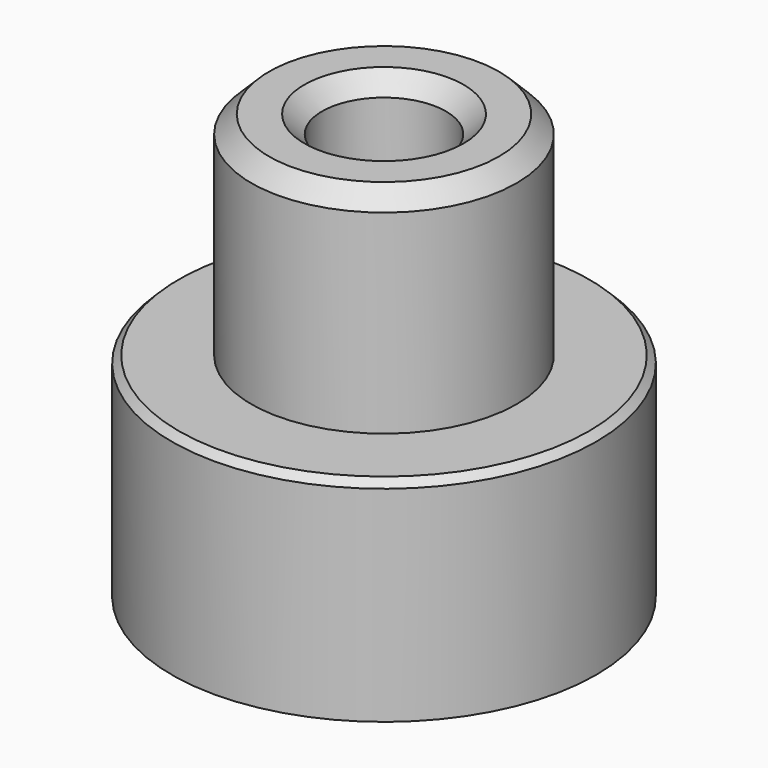
from build123d import *

# Parameters (mm, degrees)
F0_R        = 3.75
F0_R_2      = 1.75
F0_R_3      = 0.9
F1_DEPTH    = 6
F0_R_4      = 6
F1_FACE_R   = 3.75
F1_FACE_R_2 = 0.9
F2_DEPTH    = 6
F3_START    = 8
F3_DEPTH    = 6
F4_SIZE     = 0.5
F5_SIZE     = 0.2
F6_SIZE     = 0.5


with BuildPart() as f1:
    # F0 (on Top) → F1 (new body)
    with BuildSketch(Plane.XY):
        Circle(F0_R)
        Circle(F0_R_2, mode=Mode.SUBTRACT)
        Circle(F0_R_2)
        Circle(F0_R_3, mode=Mode.SUBTRACT)
    extrude(amount=F1_DEPTH)

    # F0 (on Top) + F1_face (on face) → F2 (join)
    with BuildSketch(Plane.XY):
        Circle(F0_R_4)
        Circle(F0_R, mode=Mode.SUBTRACT)
    with BuildSketch(Plane.XY.offset(6)):
        Circle(F1_FACE_R)
        Circle(F1_FACE_R_2, mode=Mode.SUBTRACT)
    extrude(amount=F2_DEPTH)

    # F0 (on Top) → F3 (cut)
    with BuildSketch(Plane.XY.offset(F3_START)):
        Circle(F0_R_2)
        Circle(F0_R_3, mode=Mode.SUBTRACT)
    extrude(amount=F3_DEPTH, mode=Mode.SUBTRACT)

    # F4
    f4_edges = [f1.edges().sort_by_distance(p)[0] for p in [
        (-0.9, 0, 0),
    ]]
    chamfer(f4_edges, length=F4_SIZE)

    # F5
    f5_edges = [f1.edges().sort_by_distance(p)[0] for p in [
        (-6, 0, 6),
    ]]
    chamfer(f5_edges, length=F5_SIZE)

    # F6
    f6_edges = [f1.edges().sort_by_distance(p)[0] for p in [
        (-3.75, 0, 12),
        (-1.75, 0, 12),
    ]]
    chamfer(f6_edges, length=F6_SIZE)


solid = f1.part
